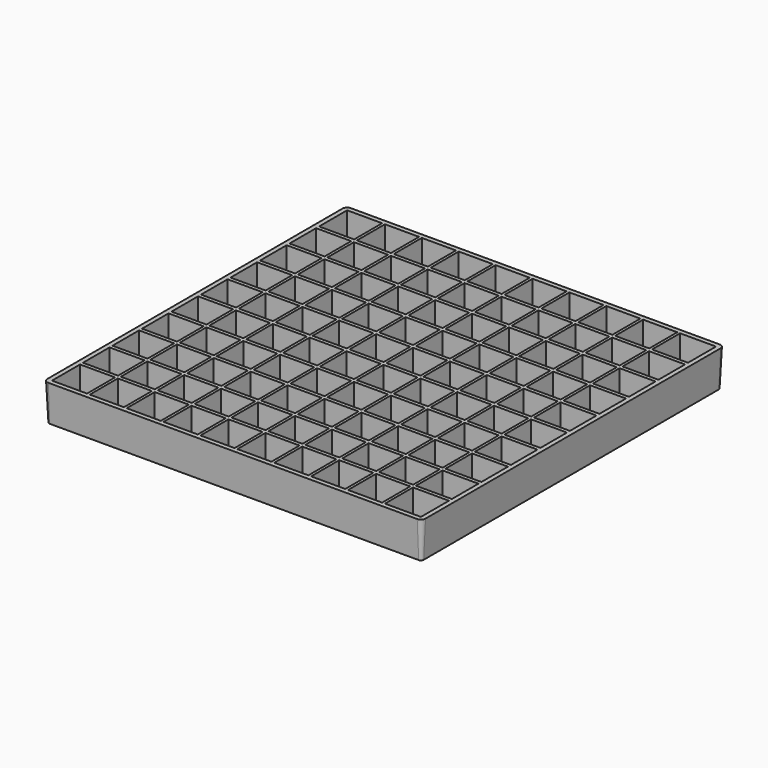
from build123d import *

# Parameters (mm, degrees)
F1_W         = 103
F1_H         = 103
F2_DEPTH     = 10
F1_W_2       = 0.75
F1_H_2       = 9
F1_H_3       = 1
F1_W_3       = 9.25
F1_H_4       = 9.5
F1_W_4       = 9.75
F1_W_5       = 9.5
F3_DEPTH     = 10
F4_R         = 1.5
F5_T1_DEPTH  = 100
F5_T3_DEPTH  = 100
F5_T6_ANGLE  = 90
F5_T8_ANGLE  = 90
F5_T10_ANGLE = 90
F5_T12_ANGLE = 90


# Not quite as in the source:
# - a fillet or chamfer that OpenCascade refuses, or shapes differently, is made with other operations: its cross-section is extruded or revolved along the edge and cut away or added


with BuildPart() as f2:
    # F1 (on Top) → F2 (new body)
    with BuildSketch(Plane.XY):
        Rectangle(F1_W, F1_H)
        Polygon((40.25, 50), (50, 50), (50, 40.5), (50, 39.5), (50, 30.5), (50, 29.5), (50, 20.5), (50, 19.5), (50, 10.5), (50, 9.5), (50, 0.5), (50, -0.5), (50, -9.5), (50, -10.5), (50, -19.5), (50, -20.5), (50, -29.5), (50, -30.5), (50, -39.5), (50, -40.5), (50, -50), (40.25, -50), (39.5, -50), (30.25, -50), (29.5, -50), (20.25, -50), (19.5, -50), (10.25, -50), (9.5, -50), (0.25, -50), (-0.5, -50), (-9.75, -50), (-10.5, -50), (-19.75, -50), (-20.5, -50), (-29.75, -50), (-30.5, -50), (-39.75, -50), (-40.5, -50), (-50, -50), (-50, -40.5), (-50, -39.5), (-50, -30.5), (-50, -29.5), (-50, -20.5), (-50, -19.5), (-50, -10.5), (-50, -9.5), (-50, -0.5), (-50, 0.5), (-50, 9.5), (-50, 10.5), (-50, 19.5), (-50, 20.5), (-50, 29.5), (-50, 30.5), (-50, 39.5), (-50, 40.5), (-50, 50), (-40.5, 50), (-39.75, 50), (-30.5, 50), (-29.75, 50), (-20.5, 50), (-19.75, 50), (-10.5, 50), (-9.75, 50), (-0.5, 50), (0.25, 50), (9.5, 50), (10.25, 50), (19.5, 50), (20.25, 50), (29.5, 50), (30.25, 50), (39.5, 50), align=None, mode=Mode.SUBTRACT)
    extrude(amount=F2_DEPTH)

    # F1 (on Top) → F3 (join)
    with BuildSketch(Plane.XY):
        with Locations((-30.125, -15)):
            Rectangle(F1_W_2, F1_H_2)
        with Locations((-30.125, -20)):
            Rectangle(F1_W_2, F1_H_3)
        with Locations((29.875, 20)):
            Rectangle(F1_W_2, F1_H_3)
        with Locations((-35.125, 0)):
            Rectangle(F1_W_3, F1_H_3)
        with Locations((-25.125, -30)):
            Rectangle(F1_W_3, F1_H_3)
        with Locations((-0.125, -5)):
            Rectangle(F1_W_2, F1_H_2)
        with Locations((-30.125, -25)):
            Rectangle(F1_W_2, F1_H_2)
        with Locations((-25.125, -10)):
            Rectangle(F1_W_3, F1_H_3)
        with Locations((-40.125, 30)):
            Rectangle(F1_W_2, F1_H_3)
        with Locations((4.875, 20)):
            Rectangle(F1_W_3, F1_H_3)
        with Locations((-25.125, 30)):
            Rectangle(F1_W_3, F1_H_3)
        with Locations((19.875, -35)):
            Rectangle(F1_W_2, F1_H_2)
        with Locations((-35.125, 30)):
            Rectangle(F1_W_3, F1_H_3)
        with Locations((39.875, 10)):
            Rectangle(F1_W_2, F1_H_3)
        with Locations((-30.125, 20)):
            Rectangle(F1_W_2, F1_H_3)
        with Locations((-20.125, -20)):
            Rectangle(F1_W_2, F1_H_3)
        with Locations((-25.125, 0)):
            Rectangle(F1_W_3, F1_H_3)
        with Locations((39.875, -15)):
            Rectangle(F1_W_2, F1_H_2)
        with Locations((24.875, 0)):
            Rectangle(F1_W_3, F1_H_3)
        with Locations((-0.125, 10)):
            Rectangle(F1_W_2, F1_H_3)
        with Locations((-5.125, -30)):
            Rectangle(F1_W_3, F1_H_3)
        with Locations((9.875, 30)):
            Rectangle(F1_W_2, F1_H_3)
        with Locations((24.875, 30)):
            Rectangle(F1_W_3, F1_H_3)
        with Locations((39.875, 40)):
            Rectangle(F1_W_2, F1_H_3)
        with Locations((34.875, 20)):
            Rectangle(F1_W_3, F1_H_3)
        with Locations((9.875, -15)):
            Rectangle(F1_W_2, F1_H_2)
        with Locations((19.875, -15)):
            Rectangle(F1_W_2, F1_H_2)
        with Locations((-40.125, 25)):
            Rectangle(F1_W_2, F1_H_2)
        with Locations((19.875, 0)):
            Rectangle(F1_W_2, F1_H_3)
        with Locations((9.875, -20)):
            Rectangle(F1_W_2, F1_H_3)
        with Locations((4.875, 40)):
            Rectangle(F1_W_3, F1_H_3)
        with Locations((-20.125, 25)):
            Rectangle(F1_W_2, F1_H_2)
        with Locations((-0.125, 30)):
            Rectangle(F1_W_2, F1_H_3)
        with Locations((-0.125, 35)):
            Rectangle(F1_W_2, F1_H_2)
        with Locations((9.875, -30)):
            Rectangle(F1_W_2, F1_H_3)
        with Locations((14.875, 30)):
            Rectangle(F1_W_3, F1_H_3)
        with Locations((9.875, -5)):
            Rectangle(F1_W_2, F1_H_2)
        with Locations((-15.125, -40)):
            Rectangle(F1_W_3, F1_H_3)
        with Locations((24.875, -20)):
            Rectangle(F1_W_3, F1_H_3)
        with Locations((-35.125, 40)):
            Rectangle(F1_W_3, F1_H_3)
        with Locations((-40.125, 15)):
            Rectangle(F1_W_2, F1_H_2)
        with Locations((19.875, 40)):
            Rectangle(F1_W_2, F1_H_3)
        with Locations((24.875, 40)):
            Rectangle(F1_W_3, F1_H_3)
        with Locations((19.875, -25)):
            Rectangle(F1_W_2, F1_H_2)
        with Locations((-5.125, -10)):
            Rectangle(F1_W_3, F1_H_3)
        with Locations((-25.125, -40)):
            Rectangle(F1_W_3, F1_H_3)
        with Locations((-30.125, -10)):
            Rectangle(F1_W_2, F1_H_3)
        with Locations((-0.125, 25)):
            Rectangle(F1_W_2, F1_H_2)
        with Locations((9.875, -35)):
            Rectangle(F1_W_2, F1_H_2)
        with Locations((39.875, -40)):
            Rectangle(F1_W_2, F1_H_3)
        with Locations((9.875, 0)):
            Rectangle(F1_W_2, F1_H_3)
        with Locations((-20.125, -25)):
            Rectangle(F1_W_2, F1_H_2)
        with Locations((-35.125, -40)):
            Rectangle(F1_W_3, F1_H_3)
        with Locations((9.875, 15)):
            Rectangle(F1_W_2, F1_H_2)
        with Locations((39.875, -5)):
            Rectangle(F1_W_2, F1_H_2)
        with Locations((24.875, -40)):
            Rectangle(F1_W_3, F1_H_3)
        with Locations((-5.125, 30)):
            Rectangle(F1_W_3, F1_H_3)
        with Locations((-10.125, -40)):
            Rectangle(F1_W_2, F1_H_3)
        with Locations((-30.125, -30)):
            Rectangle(F1_W_2, F1_H_3)
        with Locations((-20.125, -15)):
            Rectangle(F1_W_2, F1_H_2)
        with Locations((9.875, -40)):
            Rectangle(F1_W_2, F1_H_3)
        with Locations((19.875, 10)):
            Rectangle(F1_W_2, F1_H_3)
        with Locations((14.875, -20)):
            Rectangle(F1_W_3, F1_H_3)
        with Locations((9.875, 5)):
            Rectangle(F1_W_2, F1_H_2)
        with Locations((34.875, -30)):
            Rectangle(F1_W_3, F1_H_3)
        with Locations((29.875, -40)):
            Rectangle(F1_W_2, F1_H_3)
        with Locations((-5.125, 0)):
            Rectangle(F1_W_3, F1_H_3)
        with Locations((-15.125, 30)):
            Rectangle(F1_W_3, F1_H_3)
        with Locations((-30.125, 30)):
            Rectangle(F1_W_2, F1_H_3)
        with Locations((39.875, 15)):
            Rectangle(F1_W_2, F1_H_2)
        with Locations((4.875, -40)):
            Rectangle(F1_W_3, F1_H_3)
        with Locations((34.875, 40)):
            Rectangle(F1_W_3, F1_H_3)
        with Locations((-25.125, 40)):
            Rectangle(F1_W_3, F1_H_3)
        with Locations((-30.125, -5)):
            Rectangle(F1_W_2, F1_H_2)
        with Locations((-20.125, -10)):
            Rectangle(F1_W_2, F1_H_3)
        with Locations((-20.125, 5)):
            Rectangle(F1_W_2, F1_H_2)
        with Locations((14.875, 10)):
            Rectangle(F1_W_3, F1_H_3)
        with Locations((-20.125, 35)):
            Rectangle(F1_W_2, F1_H_2)
        with Locations((-30.125, 5)):
            Rectangle(F1_W_2, F1_H_2)
        with Locations((-40.125, 10)):
            Rectangle(F1_W_2, F1_H_3)
        with Locations((19.875, 20)):
            Rectangle(F1_W_2, F1_H_3)
        with Locations((24.875, -10)):
            Rectangle(F1_W_3, F1_H_3)
        with Locations((29.875, 30)):
            Rectangle(F1_W_2, F1_H_3)
        with Locations((39.875, -35)):
            Rectangle(F1_W_2, F1_H_2)
        with Locations((24.875, -30)):
            Rectangle(F1_W_3, F1_H_3)
        with Locations((9.875, 10)):
            Rectangle(F1_W_2, F1_H_3)
        with Locations((4.875, 0)):
            Rectangle(F1_W_3, F1_H_3)
        with Locations((29.875, 40)):
            Rectangle(F1_W_2, F1_H_3)
        with Locations((-15.125, 0)):
            Rectangle(F1_W_3, F1_H_3)
        with Locations((39.875, -10)):
            Rectangle(F1_W_2, F1_H_3)
        with Locations((-0.125, 5)):
            Rectangle(F1_W_2, F1_H_2)
        with Locations((14.875, -40)):
            Rectangle(F1_W_3, F1_H_3)
        with Locations((29.875, 25)):
            Rectangle(F1_W_2, F1_H_2)
        with Locations((-10.125, 0)):
            Rectangle(F1_W_2, F1_H_3)
        with Locations((-10.125, -5)):
            Rectangle(F1_W_2, F1_H_2)
        with Locations((14.875, 20)):
            Rectangle(F1_W_3, F1_H_3)
        with Locations((-0.125, 20)):
            Rectangle(F1_W_2, F1_H_3)
        with Locations((24.875, 20)):
            Rectangle(F1_W_3, F1_H_3)
        with Locations((19.875, -10)):
            Rectangle(F1_W_2, F1_H_3)
        with Locations((4.875, -20)):
            Rectangle(F1_W_3, F1_H_3)
        with Locations((-25.125, 10)):
            Rectangle(F1_W_3, F1_H_3)
        with Locations((24.875, 10)):
            Rectangle(F1_W_3, F1_H_3)
        with Locations((-15.125, 40)):
            Rectangle(F1_W_3, F1_H_3)
        with Locations((-10.125, -20)):
            Rectangle(F1_W_2, F1_H_3)
        with Locations((-5.125, -20)):
            Rectangle(F1_W_3, F1_H_3)
        with Locations((-40.125, -10)):
            Rectangle(F1_W_2, F1_H_3)
        with Locations((-40.125, 40)):
            Rectangle(F1_W_2, F1_H_3)
        with Locations((-30.125, -40)):
            Rectangle(F1_W_2, F1_H_3)
        with Locations((-25.125, 20)):
            Rectangle(F1_W_3, F1_H_3)
        with Locations((-20.125, 20)):
            Rectangle(F1_W_2, F1_H_3)
        with Locations((34.875, 10)):
            Rectangle(F1_W_3, F1_H_3)
        with Locations((19.875, 30)):
            Rectangle(F1_W_2, F1_H_3)
        with Locations((19.875, 25)):
            Rectangle(F1_W_2, F1_H_2)
        with Locations((-0.125, 15)):
            Rectangle(F1_W_2, F1_H_2)
        with Locations((9.875, -25)):
            Rectangle(F1_W_2, F1_H_2)
        with Locations((-20.125, -5)):
            Rectangle(F1_W_2, F1_H_2)
        with Locations((-40.125, -30)):
            Rectangle(F1_W_2, F1_H_3)
        with Locations((-15.125, 10)):
            Rectangle(F1_W_3, F1_H_3)
        with Locations((-20.125, 0)):
            Rectangle(F1_W_2, F1_H_3)
        with Locations((29.875, 35)):
            Rectangle(F1_W_2, F1_H_2)
        with Locations((-25.125, -20)):
            Rectangle(F1_W_3, F1_H_3)
        with Locations((-40.125, 20)):
            Rectangle(F1_W_2, F1_H_3)
        with Locations((-20.125, -40)):
            Rectangle(F1_W_2, F1_H_3)
        with Locations((-20.125, 10)):
            Rectangle(F1_W_2, F1_H_3)
        with Locations((-15.125, 20)):
            Rectangle(F1_W_3, F1_H_3)
        with Locations((-10.125, -30)):
            Rectangle(F1_W_2, F1_H_3)
        with Locations((-0.125, -35)):
            Rectangle(F1_W_2, F1_H_2)
        with Locations((9.875, 25)):
            Rectangle(F1_W_2, F1_H_2)
        with Locations((-35.125, 20)):
            Rectangle(F1_W_3, F1_H_3)
        with Locations((-0.125, -30)):
            Rectangle(F1_W_2, F1_H_3)
        with Locations((-40.125, -40)):
            Rectangle(F1_W_2, F1_H_3)
        with Locations((-40.125, -20)):
            Rectangle(F1_W_2, F1_H_3)
        with Locations((19.875, -30)):
            Rectangle(F1_W_2, F1_H_3)
        with Locations((39.875, 20)):
            Rectangle(F1_W_2, F1_H_3)
        with Locations((-40.125, 5)):
            Rectangle(F1_W_2, F1_H_2)
        with Locations((9.875, -10)):
            Rectangle(F1_W_2, F1_H_3)
        with Locations((-30.125, 40)):
            Rectangle(F1_W_2, F1_H_3)
        with Locations((29.875, 15)):
            Rectangle(F1_W_2, F1_H_2)
        with Locations((-20.125, 30)):
            Rectangle(F1_W_2, F1_H_3)
        with Locations((-40.125, -35)):
            Rectangle(F1_W_2, F1_H_2)
        with Locations((-40.125, -25)):
            Rectangle(F1_W_2, F1_H_2)
        with Locations((34.875, 30)):
            Rectangle(F1_W_3, F1_H_3)
        with Locations((-15.125, -30)):
            Rectangle(F1_W_3, F1_H_3)
        with Locations((-30.125, 25)):
            Rectangle(F1_W_2, F1_H_2)
        with Locations((9.875, 40)):
            Rectangle(F1_W_2, F1_H_3)
        with Locations((-30.125, -35)):
            Rectangle(F1_W_2, F1_H_2)
        with Locations((-40.125, -5)):
            Rectangle(F1_W_2, F1_H_2)
        with Locations((39.875, 25)):
            Rectangle(F1_W_2, F1_H_2)
        with Locations((-20.125, -35)):
            Rectangle(F1_W_2, F1_H_2)
        with Locations((4.875, -10)):
            Rectangle(F1_W_3, F1_H_3)
        with Locations((-35.125, 10)):
            Rectangle(F1_W_3, F1_H_3)
        with Locations((39.875, -30)):
            Rectangle(F1_W_2, F1_H_3)
        with Locations((4.875, 10)):
            Rectangle(F1_W_3, F1_H_3)
        with Locations((-30.125, 15)):
            Rectangle(F1_W_2, F1_H_2)
        with Locations((14.875, 0)):
            Rectangle(F1_W_3, F1_H_3)
        with Locations((29.875, 10)):
            Rectangle(F1_W_2, F1_H_3)
        with Locations((-0.125, 40)):
            Rectangle(F1_W_2, F1_H_3)
        with Locations((34.875, -10)):
            Rectangle(F1_W_3, F1_H_3)
        with Locations((14.875, -30)):
            Rectangle(F1_W_3, F1_H_3)
        with Locations((-30.125, 10)):
            Rectangle(F1_W_2, F1_H_3)
        with Locations((19.875, -40)):
            Rectangle(F1_W_2, F1_H_3)
        with Locations((-10.125, -35)):
            Rectangle(F1_W_2, F1_H_2)
        with Locations((-0.125, -10)):
            Rectangle(F1_W_2, F1_H_3)
        with Locations((19.875, 15)):
            Rectangle(F1_W_2, F1_H_2)
        with Locations((-20.125, -30)):
            Rectangle(F1_W_2, F1_H_3)
        with Locations((-40.125, -15)):
            Rectangle(F1_W_2, F1_H_2)
        with Locations((-35.125, -20)):
            Rectangle(F1_W_3, F1_H_3)
        with Locations((-5.125, 40)):
            Rectangle(F1_W_3, F1_H_3)
        with Locations((-10.125, -10)):
            Rectangle(F1_W_2, F1_H_3)
        with Locations((34.875, 0)):
            Rectangle(F1_W_3, F1_H_3)
        with Locations((9.875, 35)):
            Rectangle(F1_W_2, F1_H_2)
        with Locations((-10.125, -25)):
            Rectangle(F1_W_2, F1_H_2)
        with Locations((-5.125, -40)):
            Rectangle(F1_W_3, F1_H_3)
        with Locations((-40.125, 0)):
            Rectangle(F1_W_2, F1_H_3)
        with Locations((39.875, 30)):
            Rectangle(F1_W_2, F1_H_3)
        with Locations((39.875, 5)):
            Rectangle(F1_W_2, F1_H_2)
        with Locations((39.875, 35)):
            Rectangle(F1_W_2, F1_H_2)
        with Locations((-30.125, 0)):
            Rectangle(F1_W_2, F1_H_3)
        with Locations((14.875, 40)):
            Rectangle(F1_W_3, F1_H_3)
        with Locations((-15.125, -10)):
            Rectangle(F1_W_3, F1_H_3)
        with Locations((-5.125, 20)):
            Rectangle(F1_W_3, F1_H_3)
        with Locations((-0.125, -40)):
            Rectangle(F1_W_2, F1_H_3)
        with Locations((-5.125, 10)):
            Rectangle(F1_W_3, F1_H_3)
        with Locations((9.875, 20)):
            Rectangle(F1_W_2, F1_H_3)
        with Locations((-20.125, 15)):
            Rectangle(F1_W_2, F1_H_2)
        with Locations((19.875, -5)):
            Rectangle(F1_W_2, F1_H_2)
        with Locations((-15.125, -20)):
            Rectangle(F1_W_3, F1_H_3)
        with Locations((34.875, -20)):
            Rectangle(F1_W_3, F1_H_3)
        with Locations((-35.125, -30)):
            Rectangle(F1_W_3, F1_H_3)
        with Locations((19.875, 5)):
            Rectangle(F1_W_2, F1_H_2)
        with Locations((-10.125, -15)):
            Rectangle(F1_W_2, F1_H_2)
        with Locations((39.875, 0)):
            Rectangle(F1_W_2, F1_H_3)
        with Locations((4.875, 30)):
            Rectangle(F1_W_3, F1_H_3)
        with Locations((14.875, -10)):
            Rectangle(F1_W_3, F1_H_3)
        with Locations((39.875, -25)):
            Rectangle(F1_W_2, F1_H_2)
        with Locations((19.875, 35)):
            Rectangle(F1_W_2, F1_H_2)
        with Locations((-0.125, -25)):
            Rectangle(F1_W_2, F1_H_2)
        with Locations((4.875, -30)):
            Rectangle(F1_W_3, F1_H_3)
        with Locations((-40.125, 35)):
            Rectangle(F1_W_2, F1_H_2)
        with Locations((19.875, -20)):
            Rectangle(F1_W_2, F1_H_3)
        with Locations((39.875, -20)):
            Rectangle(F1_W_2, F1_H_3)
        with Locations((-0.125, -15)):
            Rectangle(F1_W_2, F1_H_2)
        with Locations((34.875, -40)):
            Rectangle(F1_W_3, F1_H_3)
        with Locations((-35.125, -10)):
            Rectangle(F1_W_3, F1_H_3)
        with Locations((-30.125, 35)):
            Rectangle(F1_W_2, F1_H_2)
        with Locations((-20.125, 40)):
            Rectangle(F1_W_2, F1_H_3)
        with Locations((-0.125, -20)):
            Rectangle(F1_W_2, F1_H_3)
        with Locations((29.875, 5)):
            Rectangle(F1_W_2, F1_H_2)
        with Locations((-10.125, 25)):
            Rectangle(F1_W_2, F1_H_2)
        with Locations((29.875, -30)):
            Rectangle(F1_W_2, F1_H_3)
        with Locations((29.875, -20)):
            Rectangle(F1_W_2, F1_H_3)
        with Locations((-10.125, 40)):
            Rectangle(F1_W_2, F1_H_3)
        with Locations((-10.125, 15)):
            Rectangle(F1_W_2, F1_H_2)
        with Locations((29.875, -35)):
            Rectangle(F1_W_2, F1_H_2)
        with Locations((-10.125, 30)):
            Rectangle(F1_W_2, F1_H_3)
        with Locations((-10.125, 5)):
            Rectangle(F1_W_2, F1_H_2)
        with Locations((29.875, -5)):
            Rectangle(F1_W_2, F1_H_2)
        with Locations((29.875, -10)):
            Rectangle(F1_W_2, F1_H_3)
        with Locations((-10.125, 35)):
            Rectangle(F1_W_2, F1_H_2)
        with Locations((29.875, 0)):
            Rectangle(F1_W_2, F1_H_3)
        with Locations((29.875, -25)):
            Rectangle(F1_W_2, F1_H_2)
        with Locations((-10.125, 10)):
            Rectangle(F1_W_2, F1_H_3)
        with Locations((29.875, -15)):
            Rectangle(F1_W_2, F1_H_2)
        with Locations((-10.125, 20)):
            Rectangle(F1_W_2, F1_H_3)
        with Locations((-0.125, 0)):
            Rectangle(F1_W_2, F1_H_3)
        with Locations((-20.125, -45.25)):
            Rectangle(F1_W_2, F1_H_4)
        with Locations((29.875, -45.25)):
            Rectangle(F1_W_2, F1_H_4)
        with Locations((9.875, -45.25)):
            Rectangle(F1_W_2, F1_H_4)
        with Locations((-40.125, -45.25)):
            Rectangle(F1_W_2, F1_H_4)
        with Locations((-10.125, -45.25)):
            Rectangle(F1_W_2, F1_H_4)
        with Locations((39.875, -45.25)):
            Rectangle(F1_W_2, F1_H_4)
        with Locations((-30.125, -45.25)):
            Rectangle(F1_W_2, F1_H_4)
        with Locations((19.875, -45.25)):
            Rectangle(F1_W_2, F1_H_4)
        with Locations((-0.125, -45.25)):
            Rectangle(F1_W_2, F1_H_4)
        with Locations((45.125, -40)):
            Rectangle(F1_W_4, F1_H_3)
        with Locations((45.125, -30)):
            Rectangle(F1_W_4, F1_H_3)
        with Locations((45.125, -20)):
            Rectangle(F1_W_4, F1_H_3)
        with Locations((45.125, -10)):
            Rectangle(F1_W_4, F1_H_3)
        with Locations((45.125, 0)):
            Rectangle(F1_W_4, F1_H_3)
        with Locations((45.125, 10)):
            Rectangle(F1_W_4, F1_H_3)
        with Locations((45.125, 20)):
            Rectangle(F1_W_4, F1_H_3)
        with Locations((-45.25, -40)):
            Rectangle(F1_W_5, F1_H_3)
        with Locations((-45.25, -30)):
            Rectangle(F1_W_5, F1_H_3)
        with Locations((-45.25, -10)):
            Rectangle(F1_W_5, F1_H_3)
        with Locations((-45.25, 0)):
            Rectangle(F1_W_5, F1_H_3)
        with Locations((-45.25, 10)):
            Rectangle(F1_W_5, F1_H_3)
        with Locations((-45.25, 20)):
            Rectangle(F1_W_5, F1_H_3)
        with Locations((45.125, 30)):
            Rectangle(F1_W_4, F1_H_3)
        with Locations((45.125, 40)):
            Rectangle(F1_W_4, F1_H_3)
        with Locations((39.875, 45.25)):
            Rectangle(F1_W_2, F1_H_4)
        with Locations((29.875, 45.25)):
            Rectangle(F1_W_2, F1_H_4)
        with Locations((19.875, 45.25)):
            Rectangle(F1_W_2, F1_H_4)
        with Locations((9.875, 45.25)):
            Rectangle(F1_W_2, F1_H_4)
        with Locations((-0.125, 45.25)):
            Rectangle(F1_W_2, F1_H_4)
        with Locations((-10.125, 45.25)):
            Rectangle(F1_W_2, F1_H_4)
        with Locations((-20.125, 45.25)):
            Rectangle(F1_W_2, F1_H_4)
        with Locations((-30.125, 45.25)):
            Rectangle(F1_W_2, F1_H_4)
        with Locations((-40.125, 45.25)):
            Rectangle(F1_W_2, F1_H_4)
        with Locations((-45.25, 40)):
            Rectangle(F1_W_5, F1_H_3)
        with Locations((-45.25, 30)):
            Rectangle(F1_W_5, F1_H_3)
        with Locations((-45.25, -20)):
            Rectangle(F1_W_5, F1_H_3)
    extrude(amount=F3_DEPTH)

    # F4
    f4_edges = [f2.edges().sort_by_distance(p)[0] for p in [
        (51.5, -51.5, 5),
        (-51.5, -51.5, 5),
        (-51.5, 51.5, 5),
        (51.5, 51.5, 5),
    ]]
    fillet(f4_edges, radius=F4_R)

    # F5: chamfer of 0.75 x 15 on 1 edges, made by hand

    # F5_s2 → F5_t1 (cut)
    with BuildSketch(Plane.YZ.offset(-50)):
        Polygon((51.5, 15), (50.75, 0), (51.5, 0), align=None)
        Polygon((-50.75, 0), (-51.5, 15), (-51.5, 0), align=None)
    extrude(amount=F5_T1_DEPTH, mode=Mode.SUBTRACT)

    # F5_s4 → F5_t3 (cut)
    with BuildSketch(Plane.XZ.offset(-50)):
        Polygon((-50.75, 0), (-51.5, 15), (-51.5, 0), align=None)
        Polygon((50.75, 0), (51.5, 15), (51.5, 0), align=None)
    extrude(amount=F5_T3_DEPTH, mode=Mode.SUBTRACT)

    # F5_s5 → F5_t6 (revolve, cut)
    with BuildSketch(Plane.YZ.offset(50)):
        Polygon((50.75, 0), (51.5, 15), (51.5, 0), align=None)
    revolve(axis=Axis((50, 50, 0), (0, 0, -1)), revolution_arc=F5_T6_ANGLE, mode=Mode.SUBTRACT)

    # F5_s7 → F5_t8 (revolve, cut)
    with BuildSketch(Plane.YZ.offset(-50)):
        Polygon((50.75, 0), (51.5, 15), (51.5, 0), align=None)
    revolve(axis=Axis((-50, 50, 0), (0, 0, 1)), revolution_arc=F5_T8_ANGLE, mode=Mode.SUBTRACT)

    # F5_s9 → F5_t10 (revolve, cut)
    with BuildSketch(Plane.XZ.offset(50)):
        Polygon((-50.75, 0), (-51.5, 15), (-51.5, 0), align=None)
    revolve(axis=Axis((-50, -50, 0), (0, 0, 1)), revolution_arc=F5_T10_ANGLE, mode=Mode.SUBTRACT)

    # F5_s11 → F5_t12 (revolve, cut)
    with BuildSketch(Plane.XZ.offset(50)):
        Polygon((50.75, 0), (51.5, 15), (51.5, 0), align=None)
    revolve(axis=Axis((50, -50, 0), (0, 0, -1)), revolution_arc=F5_T12_ANGLE, mode=Mode.SUBTRACT)


solid = f2.part
